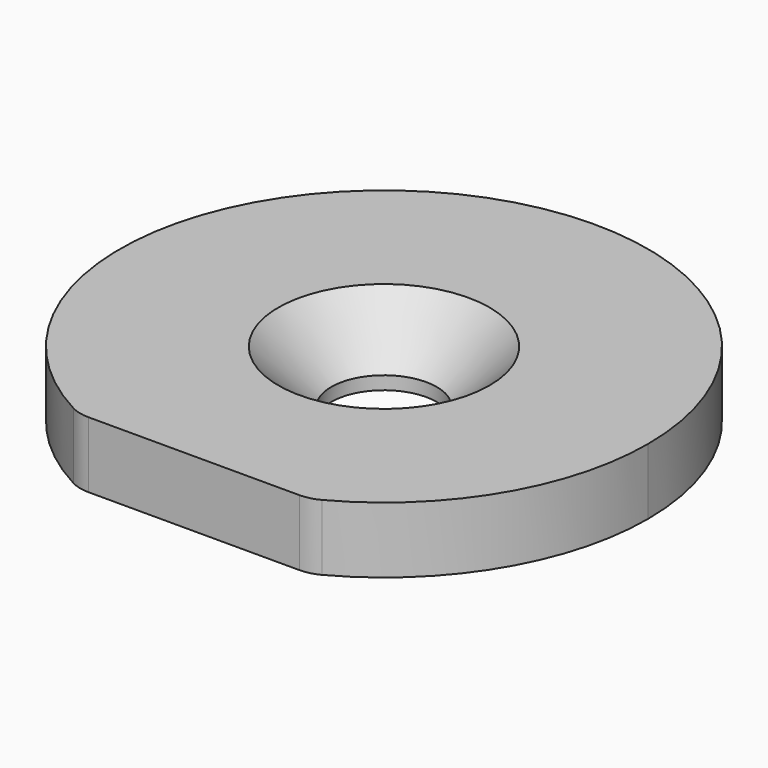
from build123d import *

# Parameters (mm, degrees)
F0_R     = 2.54
F1_DEPTH = 3.175
F2_SIZE2 = 2.54
F2_SIZE  = 2.54
F3_R     = 1.905


with BuildPart() as f1:
    # F0 (on Top) → F1 (new body)
    with BuildSketch(Plane.XY):
        with BuildLine():
            ThreePointArc((5.5358016583, -11.43), (10.7609172718, -6.7448246434), (12.7, 0))
            ThreePointArc((12.7, 0), (-6.7448246434, 10.7609172718), (-5.5358016583, -11.43))
            Line((-5.5358016583, -11.43), (5.5358016583, -11.43))
        make_face()
        Circle(F0_R, mode=Mode.SUBTRACT)
    extrude(amount=F1_DEPTH)

    # F2
    f2_edges = [f1.edges().sort_by_distance(p)[0] for p in [
        (-2.54, 0, 3.175),
    ]]
    chamfer(f2_edges, length=F2_SIZE, length2=F2_SIZE2)

    # F3
    f3_edges = [f1.edges().sort_by_distance(p)[0] for p in [
        (-5.535802, -11.43, 1.5875),
        (5.535802, -11.43, 1.5875),
    ]]
    fillet(f3_edges, radius=F3_R)


solid = f1.part
